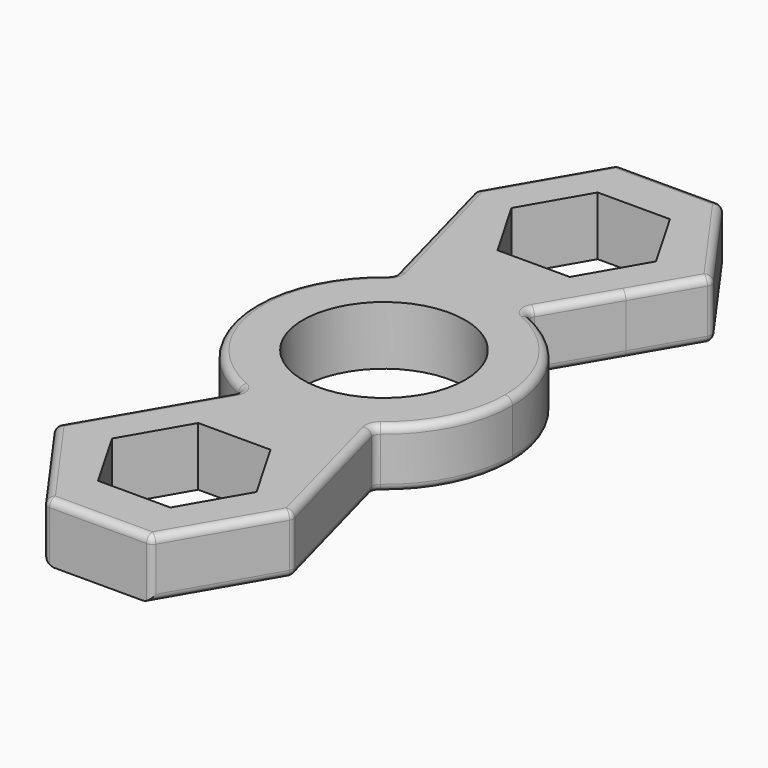
from build123d import *

# Parameters (mm, degrees)
F0_R     = 11.05
F1_DEPTH = 8
F2_COUNT = 2
F3_F1_R  = 1
F3_F2_R  = 1


with BuildPart() as f1:
    # F0 (on Top) → F1 (new body)
    with BuildSketch(Plane.XY):
        with BuildLine():
            ThreePointArc((-10.0903869269, 14.2980450295), (-8.0519633873, -15.5375636961), (17.5, 0))
            ThreePointArc((17.5, 0), (14.3285222663, 10.0470617428), (5.9636057526, 16.4525197592))
            ThreePointArc((5.9636057526, 16.4525197592), (-2.3276642918, 17.3445086106), (-10.0903869269, 14.2980450295))
        make_face()
        Circle(F0_R, mode=Mode.SUBTRACT)
        with BuildLine():
            ThreePointArc((-10.0903869269, 14.2980450295), (-2.3276642918, 17.3445086106), (5.9636057526, 16.4525197592))
            Line((5.9636057526, 16.4525197592), (11.7946313694, 26.4485646039))
            Line((11.7946313694, 26.4485646039), (16.7984124273, 35.0264757872))
            Line((16.7984124273, 35.0264757872), (6.7908498459, 49.0847229958))
            Line((6.7908498459, 49.0847229958), (-7.5056743808, 49.0847229958))
            Line((-7.5056743808, 49.0847229958), (-15.6662040079, 35.0410211056))
            Line((-15.6662040079, 35.0410211056), (-10.0903869269, 14.2980450295))
        make_face()
        Polygon((-4.9219110448, 42.525), (4.9219110448, 42.525), (9.8438220897, 34), (4.9219110448, 25.475), (-4.9219110448, 25.475), (-9.8438220897, 34), align=None, mode=Mode.SUBTRACT)
    extrude(amount=F1_DEPTH)

    # F2: F1 ×2 about axis
    f2_axis = Axis((0, 0, 0), (0, 0, 1))


with BuildPart() as f1_1:
    add(f1.part)
    for i in range(1, F2_COUNT):
        add(f1.part.rotate(f2_axis, i * 360 / F2_COUNT))

    # F3: fillet of radius 1 on 31 edges, made by hand

    # F3_f1
    f3_f1_edges = [f1_1.edges().sort_by_distance(p)[0] for p in [
        (10.0903869269, -14.2980450295, 4),
        (5.9636057526, 16.4525197592, 4),
        (-10.0903869269, 14.2980450295, 4),
        (-5.9636057526, -16.4525197592, 4),
    ]]
    fillet(f3_f1_edges, radius=F3_F1_R)

    # F3_f2
    f3_f2_edges = [f1_1.edges().sort_by_distance(p)[0] for p in [
        (7.5056743808, -49.0847229958, 4),
        (15.6662040079, -35.0410211056, 4),
        (11.5859391943, -42.0628720507, 0),
        (11.5859391943, -42.0628720507, 8),
        (12.9670524021, -24.9997237726, 0),
        (12.9670524021, -24.9997237726, 8),
        (16.7984124273, 35.0264757872, 4),
        (11.6731868984, 26.2403740629, 0),
        (11.6731868984, 26.2403740629, 8),
        (6.7908498459, 49.0847229958, 4),
        (11.7946311366, 42.0555993915, 0),
        (11.7946311366, 42.0555993915, 8),
        (-7.5056743808, 49.0847229958, 4),
        (-0.3574122675, 49.0847229958, 0),
        (-0.3574122675, 49.0847229958, 8),
        (-15.6662040079, 35.0410211056, 4),
        (-11.5859391943, 42.0628720507, 0),
        (-11.5859391943, 42.0628720507, 8),
        (-12.9670524021, 24.9997237726, 0),
        (-12.9670524021, 24.9997237726, 8),
        (-16.7984124273, -35.0264757872, 4),
        (-11.6731868984, -26.2403740629, 0),
        (-11.6731868984, -26.2403740629, 8),
        (-6.7908498459, -49.0847229958, 4),
        (-11.7946311366, -42.0555993915, 0),
        (-11.7946311366, -42.0555993915, 8),
        (0.3574122675, -49.0847229958, 8),
        (-6.4610233416, -16.640341221, 8),
        (-6.4610233416, -16.640341221, 0),
        (-10.2868728829, 14.376857273, 8),
        (-10.2868728829, 14.376857273, 0),
        (6.4610233416, 16.640341221, 8),
        (6.4610233416, 16.640341221, 0),
        (10.2868728829, -14.376857273, 8),
        (10.2868728829, -14.376857273, 0),
    ]]
    fillet(f3_f2_edges, radius=F3_F2_R)


solid = f1_1.part
